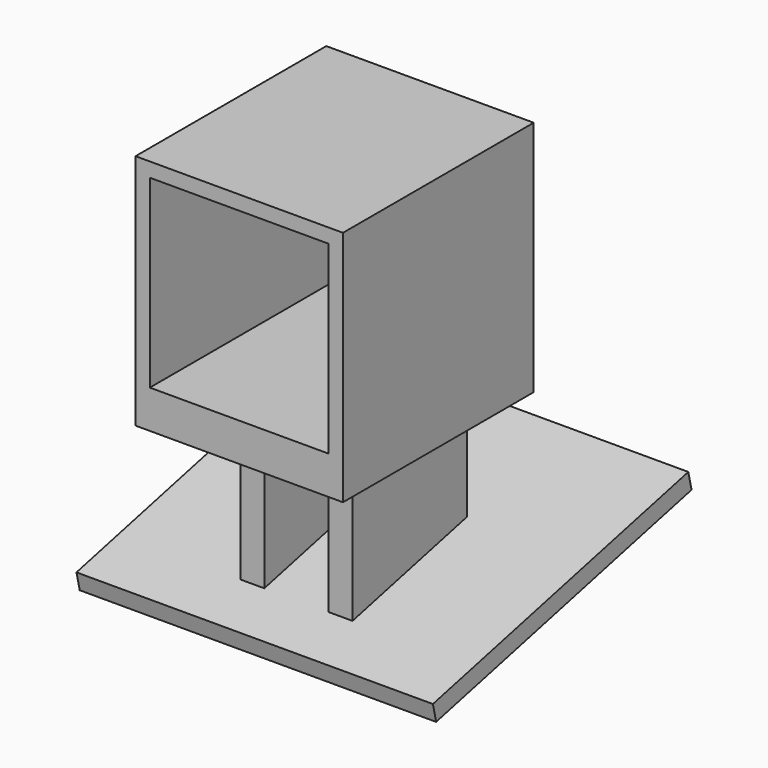
from build123d import *

# Parameters (mm, degrees)
F0_W     = 34.8
F0_H     = 39.8
F0_W_2   = 30
F0_H_2   = 35
F1_DEPTH = 40
F2_W     = 4
F2_H     = 24
F3_DEPTH = 25
F5_DEPTH = 25
F6_DEPTH = 4
F7_W     = 59.8
F7_H     = 55
F7_W_2   = 4
F7_H_2   = 24.645994744
F8_DEPTH = 3


with BuildPart() as f1:
    # F0 (on Front) → F1 (new body)
    with BuildSketch(Plane.XZ):
        with Locations((-15, 17.5)):
            Rectangle(F0_W, F0_H)
        with Locations((-15, 17.5)):
            Rectangle(F0_W_2, F0_H_2, mode=Mode.SUBTRACT)
    extrude(amount=F1_DEPTH)

    # F2 (on face) → F3 (join)
    with BuildSketch(Plane(origin=(0, 0, -2.4), x_dir=(1, 0, 0), z_dir=(0, 0, -1))):
        with Locations((-22.4, 16)):
            Rectangle(F2_W, F2_H)
        with Locations((-7.6, 16)):
            Rectangle(F2_W, F2_H)
    extrude(amount=F3_DEPTH)

    # F4 (on face) → F5 (cut)
    with BuildSketch(Plane(origin=(-24.4, 0, 0), x_dir=(0, -1, 0), z_dir=(-1, 0, 0))):
        Polygon((4, -27.4), (28, -27.4), (4, -21.7941943556), align=None)
    extrude(amount=-F5_DEPTH, mode=Mode.SUBTRACT)

    # F6 (add): a face of the model
    f6_faces = [f1.faces().sort_by_distance(p)[0] for p in [
        (-15, -20, 0),
    ]]
    extrude(f6_faces, amount=F6_DEPTH)


with BuildPart() as f8:
    # F7 (on face) → F8 (new body)
    with BuildSketch(Plane(origin=(0, 4.6202838785, -19.7807095213), x_dir=(1, 0, 0), z_dir=(0, 0.2274530082, -0.9737890578))):
        with Locations((-15, 14.9983060425)):
            Rectangle(F7_W, F7_H)
        with Locations((-22.4, 21.1753086704)):
            Rectangle(F7_W_2, F7_H_2, mode=Mode.SUBTRACT)
        with Locations((-22.4, 21.1753086704)):
            Rectangle(F7_W_2, F7_H_2)
    extrude(amount=F8_DEPTH)


solid = Compound([f1.part, f8.part])
